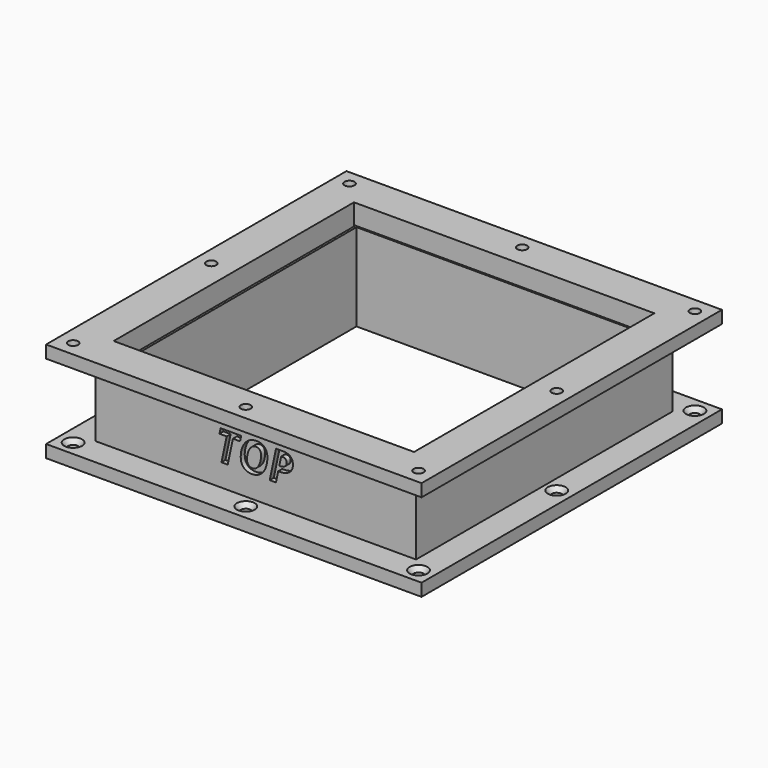
from build123d import *

# Parameters (mm, degrees)
F0_W            = 150
F0_H            = 150
F0_W_2          = 110
F0_H_2          = 110
F1_DEPTH        = 5
F2_W            = 118
F2_H            = 118
F2_W_2          = 110
F2_H_2          = 110
F3_DEPTH        = 30
F4_W            = 128
F4_H            = 128
F4_W_2          = 120
F4_H_2          = 120
F5_DEPTH        = 30
F6_W            = 150
F6_H            = 150
F6_W_2          = 120
F6_H_2          = 120
F7_DEPTH        = 5
F9_D            = 3.9624
F9_CSINK_D      = 7.1374
F9_CSINK_ANGLE  = 82
F10_TEXT_SIZE   = 16.6666666667
F11_DEPTH       = 2
F13_D           = 3.9624
F13_CSINK_D     = 7.1374
F13_CSINK_ANGLE = 82
F14_TEXT_SIZE   = 16.6666666667
F15_DEPTH       = 2
F16_T1_DEPTH    = 143
F16_T3_DEPTH    = 143
F17_T1_DEPTH    = 120
F17_T3_DEPTH    = 120
F17_T9_DEPTH    = 132.5
F17_T15_DEPTH   = 132.5
F17_T24_DEPTH   = 132.5
F17_T30_DEPTH   = 132.5
F17_T39_DEPTH   = 132.5
F17_T45_DEPTH   = 132.5
F17_T54_DEPTH   = 132.5
F17_T60_DEPTH   = 132.5


# Not quite as in the source:
# - a fillet or chamfer that OpenCascade refuses, or shapes differently, is made with other operations: its cross-section is extruded or revolved along the edge and cut away or added
# - Text() gives the source's letters only with a copy of the font that has no kerning and outlines rounded to 1/6400 em; it was checked with that copy


with BuildPart() as f1:
    # F0 (on Top) → F1 (new body)
    with BuildSketch(Plane.XY):
        Rectangle(F0_W, F0_H)
        Rectangle(F0_W_2, F0_H_2, mode=Mode.SUBTRACT)
    extrude(amount=F1_DEPTH)

    # F2 (on face) → F3 (join)
    with BuildSketch(Plane.XY.offset(5)):
        Rectangle(F2_W, F2_H)
        Rectangle(F2_W_2, F2_H_2, mode=Mode.SUBTRACT)
    extrude(amount=F3_DEPTH)

    # F9 (through all)
    with Locations(Plane.XY.offset(5)):
        with Locations((-69, 69), (69, 69), (69, -69), (-69, -69), (-69, 0), (0, 69), (0, -69), (69, 0)):
            CounterSinkHole(F9_D / 2, F9_CSINK_D / 2, counter_sink_angle=F9_CSINK_ANGLE)

    # F10 (on face) → F11 (cut)
    with BuildSketch(Plane.XZ.offset(59)):
        with Locations((-34.0950520833, 14)):
            Text('BOTTOM', F10_TEXT_SIZE, font='Open Sans', font_style=FontStyle.BOLDITALIC, text_align=(TextAlign.LEFT, TextAlign.BOTTOM))
    extrude(amount=-F11_DEPTH, mode=Mode.SUBTRACT)

    # F16: fillet of radius 5 on 4 edges, made by hand

    # F16_s2 → F16_t1 (cut)
    with BuildSketch(Plane.YZ.offset(-71.5)):
        with BuildLine():
            ThreePointArc((-59, 30), (-57.5355339059, 33.5355339059), (-54, 35))
            Line((-54, 35), (-59, 35))
            Line((-59, 35), (-59, 30))
        make_face()
        with BuildLine():
            ThreePointArc((59, 30), (57.5355339059, 33.5355339059), (54, 35))
            Line((54, 35), (59, 35))
            Line((59, 35), (59, 30))
        make_face()
    extrude(amount=F16_T1_DEPTH, mode=Mode.SUBTRACT)

    # F16_s4 → F16_t3 (cut)
    with BuildSketch(Plane.XZ.offset(-71.5)):
        with BuildLine():
            ThreePointArc((-59, 30), (-57.5355339059, 33.5355339059), (-54, 35))
            Line((-54, 35), (-59, 35))
            Line((-59, 35), (-59, 30))
        make_face()
        with BuildLine():
            ThreePointArc((59, 30), (57.5355339059, 33.5355339059), (54, 35))
            Line((54, 35), (59, 35))
            Line((59, 35), (59, 30))
        make_face()
    extrude(amount=F16_T3_DEPTH, mode=Mode.SUBTRACT)


with BuildPart() as f5:
    # F4 (on face) → F5 (new body)
    with BuildSketch(Plane.XY.offset(35)):
        Rectangle(F4_W, F4_H)
        Rectangle(F4_W_2, F4_H_2, mode=Mode.SUBTRACT)
    extrude(amount=-F5_DEPTH)

    # F6 (on face) → F7 (join)
    with BuildSketch(Plane.XY.offset(35)):
        Rectangle(F6_W, F6_H)
        Rectangle(F6_W_2, F6_H_2, mode=Mode.SUBTRACT)
    extrude(amount=F7_DEPTH)

    # F13 (through all)
    with Locations(Plane(origin=(0, 0, 35), x_dir=(1, 0, 0), z_dir=(0, 0, -1))):
        with Locations((-69, 69), (0, 69), (69, 69), (69, 0), (69, -69), (0, -69), (-69, -69), (-69, 0)):
            CounterSinkHole(F13_D / 2, F13_CSINK_D / 2, counter_sink_angle=F13_CSINK_ANGLE)

    # F14 (on face) → F15 (cut)
    with BuildSketch(Plane.XZ.offset(64)):
        with Locations((-15.8893229167, 14)):
            Text('TOP', F14_TEXT_SIZE, font='Open Sans', font_style=FontStyle.BOLDITALIC, text_align=(TextAlign.LEFT, TextAlign.BOTTOM))
    extrude(amount=-F15_DEPTH, mode=Mode.SUBTRACT)

    # F17: fillet of radius 5 on 4 edges, made by hand

    # F17_s2 → F17_t1 (cut)
    with BuildSketch(Plane.YZ.offset(-60)):
        with BuildLine():
            ThreePointArc((-65, 5), (-61.4644660941, 6.4644660941), (-60, 10))
            Line((-60, 10), (-60, 5))
            Line((-60, 5), (-65, 5))
        make_face()
        with BuildLine():
            ThreePointArc((65, 5), (61.4644660941, 6.4644660941), (60, 10))
            Line((60, 10), (60, 5))
            Line((60, 5), (65, 5))
        make_face()
    extrude(amount=F17_T1_DEPTH, mode=Mode.SUBTRACT)

    # F17_s4 → F17_t3 (cut)
    with BuildSketch(Plane.XZ.offset(-60)):
        with BuildLine():
            ThreePointArc((-65, 5), (-61.4644660941, 6.4644660941), (-60, 10))
            Line((-60, 10), (-60, 5))
            Line((-60, 5), (-65, 5))
        make_face()
        with BuildLine():
            ThreePointArc((65, 5), (61.4644660941, 6.4644660941), (60, 10))
            Line((60, 10), (60, 5))
            Line((60, 5), (65, 5))
        make_face()
    extrude(amount=F17_T3_DEPTH, mode=Mode.SUBTRACT)


with BuildPart() as f17_tool7:
    # F17_s8 → F17_t9 (new body)
    with BuildSketch(Plane.YZ.offset(72.5)):
        with BuildLine():
            ThreePointArc((-65, 5), (-61.4644660941, 6.4644660941), (-60, 10))
            Line((-60, 10), (-60, 5))
            Line((-60, 5), (-65, 5))
        make_face()
    extrude(amount=-F17_T9_DEPTH)

    split(bisect_by=Plane.YZ.offset(64), keep=Keep.BOTTOM)

    split(bisect_by=Plane.XZ.offset(64), keep=Keep.BOTTOM)

    split(bisect_by=Plane.YZ.offset(60), keep=Keep.TOP)


with BuildPart() as f17_tool13:
    # F17_s14 → F17_t15 (new body)
    with BuildSketch(Plane.XZ.offset(-60)):
        with BuildLine():
            ThreePointArc((65, 5), (61.4644660941, 6.4644660941), (60, 10))
            Line((60, 10), (60, 5))
            Line((60, 5), (65, 5))
        make_face()
    extrude(amount=F17_T15_DEPTH)

    split(bisect_by=Plane.YZ.offset(64), keep=Keep.BOTTOM)

    split(bisect_by=Plane.XZ.offset(64), keep=Keep.BOTTOM)

    split(bisect_by=Plane.XZ.offset(60), keep=Keep.TOP)


with BuildPart() as f17_tool7_1:
    add(f17_tool7.part)

    # F17_t19: intersect F17_tool13
    add(f17_tool13.part, mode=Mode.INTERSECT)


with BuildPart() as f5_1:
    add(f5.part)

    # F17_t5: cut F17_tool7
    add(f17_tool7_1.part, mode=Mode.SUBTRACT)


with BuildPart() as f17_tool22:
    # F17_s23 → F17_t24 (new body)
    with BuildSketch(Plane.YZ.offset(60)):
        with BuildLine():
            ThreePointArc((-65, 5), (-61.4644660941, 6.4644660941), (-60, 10))
            Line((-60, 10), (-60, 5))
            Line((-60, 5), (-65, 5))
        make_face()
    extrude(amount=-F17_T24_DEPTH)

    split(bisect_by=Plane.YZ.offset(-64), keep=Keep.TOP)

    split(bisect_by=Plane.XZ.offset(64), keep=Keep.BOTTOM)

    split(bisect_by=Plane.YZ.offset(-60), keep=Keep.BOTTOM)


with BuildPart() as f17_tool28:
    # F17_s29 → F17_t30 (new body)
    with BuildSketch(Plane.XZ.offset(72.5)):
        with BuildLine():
            ThreePointArc((-65, 5), (-61.4644660941, 6.4644660941), (-60, 10))
            Line((-60, 10), (-60, 5))
            Line((-60, 5), (-65, 5))
        make_face()
    extrude(amount=-F17_T30_DEPTH)

    split(bisect_by=Plane.YZ.offset(-64), keep=Keep.TOP)

    split(bisect_by=Plane.XZ.offset(64), keep=Keep.BOTTOM)

    split(bisect_by=Plane.XZ.offset(60), keep=Keep.TOP)


with BuildPart() as f17_tool22_1:
    add(f17_tool22.part)

    # F17_t34: intersect F17_tool28
    add(f17_tool28.part, mode=Mode.INTERSECT)


with BuildPart() as f5_2:
    add(f5_1.part)

    # F17_t20: cut F17_tool22
    add(f17_tool22_1.part, mode=Mode.SUBTRACT)


with BuildPart() as f17_tool37:
    # F17_s38 → F17_t39 (new body)
    with BuildSketch(Plane.XZ.offset(60)):
        with BuildLine():
            ThreePointArc((-65, 5), (-61.4644660941, 6.4644660941), (-60, 10))
            Line((-60, 10), (-60, 5))
            Line((-60, 5), (-65, 5))
        make_face()
    extrude(amount=-F17_T39_DEPTH)

    split(bisect_by=Plane.XZ.offset(-64), keep=Keep.TOP)

    split(bisect_by=Plane.YZ.offset(-64), keep=Keep.TOP)

    split(bisect_by=Plane.XZ.offset(-60), keep=Keep.BOTTOM)


with BuildPart() as f17_tool43:
    # F17_s44 → F17_t45 (new body)
    with BuildSketch(Plane.YZ.offset(-72.5)):
        with BuildLine():
            ThreePointArc((65, 5), (61.4644660941, 6.4644660941), (60, 10))
            Line((60, 10), (60, 5))
            Line((60, 5), (65, 5))
        make_face()
    extrude(amount=F17_T45_DEPTH)

    split(bisect_by=Plane.XZ.offset(-64), keep=Keep.TOP)

    split(bisect_by=Plane.YZ.offset(-64), keep=Keep.TOP)

    split(bisect_by=Plane.YZ.offset(-60), keep=Keep.BOTTOM)


with BuildPart() as f17_tool37_1:
    add(f17_tool37.part)

    # F17_t49: intersect F17_tool43
    add(f17_tool43.part, mode=Mode.INTERSECT)


with BuildPart() as f5_3:
    add(f5_2.part)

    # F17_t35: cut F17_tool37
    add(f17_tool37_1.part, mode=Mode.SUBTRACT)


with BuildPart() as f17_tool52:
    # F17_s53 → F17_t54 (new body)
    with BuildSketch(Plane.YZ.offset(-60)):
        with BuildLine():
            ThreePointArc((65, 5), (61.4644660941, 6.4644660941), (60, 10))
            Line((60, 10), (60, 5))
            Line((60, 5), (65, 5))
        make_face()
    extrude(amount=F17_T54_DEPTH)

    split(bisect_by=Plane.XZ.offset(-64), keep=Keep.TOP)

    split(bisect_by=Plane.YZ.offset(64), keep=Keep.BOTTOM)

    split(bisect_by=Plane.YZ.offset(60), keep=Keep.TOP)


with BuildPart() as f17_tool58:
    # F17_s59 → F17_t60 (new body)
    with BuildSketch(Plane.XZ.offset(-72.5)):
        with BuildLine():
            ThreePointArc((65, 5), (61.4644660941, 6.4644660941), (60, 10))
            Line((60, 10), (60, 5))
            Line((60, 5), (65, 5))
        make_face()
    extrude(amount=F17_T60_DEPTH)

    split(bisect_by=Plane.XZ.offset(-64), keep=Keep.TOP)

    split(bisect_by=Plane.YZ.offset(64), keep=Keep.BOTTOM)

    split(bisect_by=Plane.XZ.offset(-60), keep=Keep.BOTTOM)


with BuildPart() as f17_tool52_1:
    add(f17_tool52.part)

    # F17_t64: intersect F17_tool58
    add(f17_tool58.part, mode=Mode.INTERSECT)


with BuildPart() as f5_4:
    add(f5_3.part)

    # F17_t50: cut F17_tool52
    add(f17_tool52_1.part, mode=Mode.SUBTRACT)


solid = Compound([f1.part, f5_4.part])
